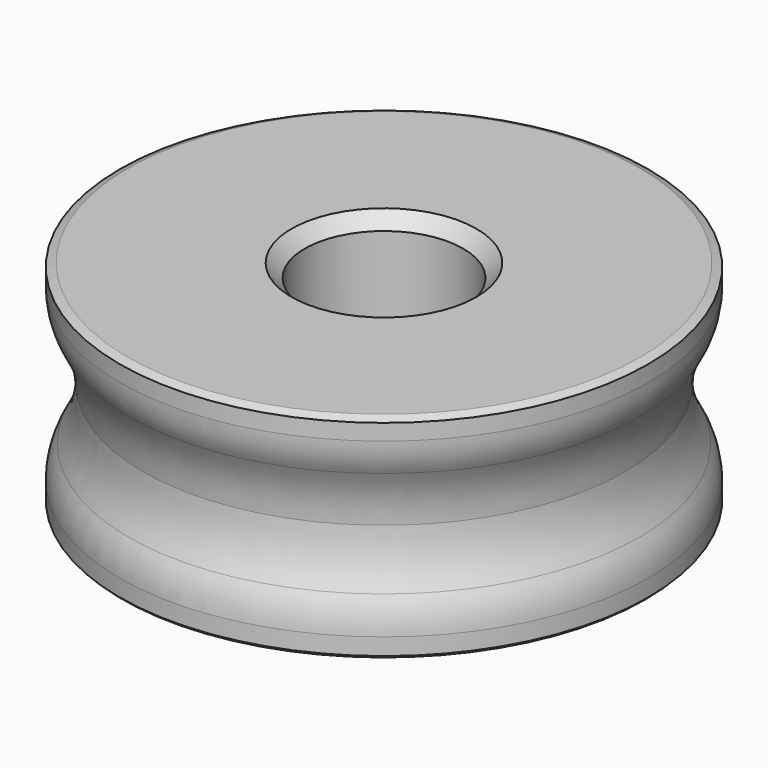
from build123d import *

# Parameters (mm, degrees)
F2_SIZE = 0.1


# Not quite as in the source:
# - a fillet or chamfer that OpenCascade refuses, or shapes differently, is made with other operations: its cross-section is extruded or revolved along the edge and cut away or added


with BuildPart() as f1:
    # F0 (on Front) → F1 (revolve)
    with BuildSketch(Plane.XZ):
        with BuildLine():
            Line((10, 4), (3, 4))
            Line((3, 4), (3, 0))
            Line((3, 0), (3, -4))
            Line((3, -4), (10, -4))
            Line((10, -4), (10, -3.2615188186))
            ThreePointArc((10, -3.2615188186), (9.9141508898, -2.6119993954), (9.6624996151, -2.0070885037))
            ThreePointArc((9.6624996151, -2.0070885037), (9.2598575755, -1.0392310772), (9.1224989992, 0))
            ThreePointArc((9.1224989992, 0), (9.2598575755, 1.0392310772), (9.6624996151, 2.0070885037))
            ThreePointArc((9.6624996151, 2.0070885037), (9.9141508898, 2.6119993954), (10, 3.2615188186))
            Line((10, 3.2615188186), (10, 4))
        make_face()
    revolve(axis=Axis((0, 0, 5.2388195913), (0, 0, 1)))

    # F2
    f2_edges = [f1.edges().sort_by_distance(p)[0] for p in [
        (-10, 0, 4),
        (-10, 0, -4),
    ]]
    chamfer(f2_edges, length=F2_SIZE)

    # F3: chamfer of 0.5 on 3 edges, made by hand

    # F3_s1 → F3_t2 (revolve, cut)
    with BuildSketch(Plane.XZ):
        Polygon((3.5, 4), (3, 3.5), (3, 4), align=None)
    revolve(axis=Axis((0, 0, 4), (0, 0, 1)), mode=Mode.SUBTRACT)

    # F3_s3 → F3_t4 (revolve, cut)
    with BuildSketch(Plane.XZ):
        Polygon((3, -3.5), (3.5, -4), (3, -4), align=None)
    revolve(axis=Axis((0, 0, -4), (0, 0, 1)), mode=Mode.SUBTRACT)

    # F3_s5 → F3_t6 (revolve, cut)
    with BuildSketch(Plane.XZ):
        Polygon((10.0464466094, 3.8535533906), (9.6928932188, 4), (9.9, 4), align=None)
    revolve(axis=Axis((0, 0, 4), (0, 0, 1)), mode=Mode.SUBTRACT)


solid = f1.part
